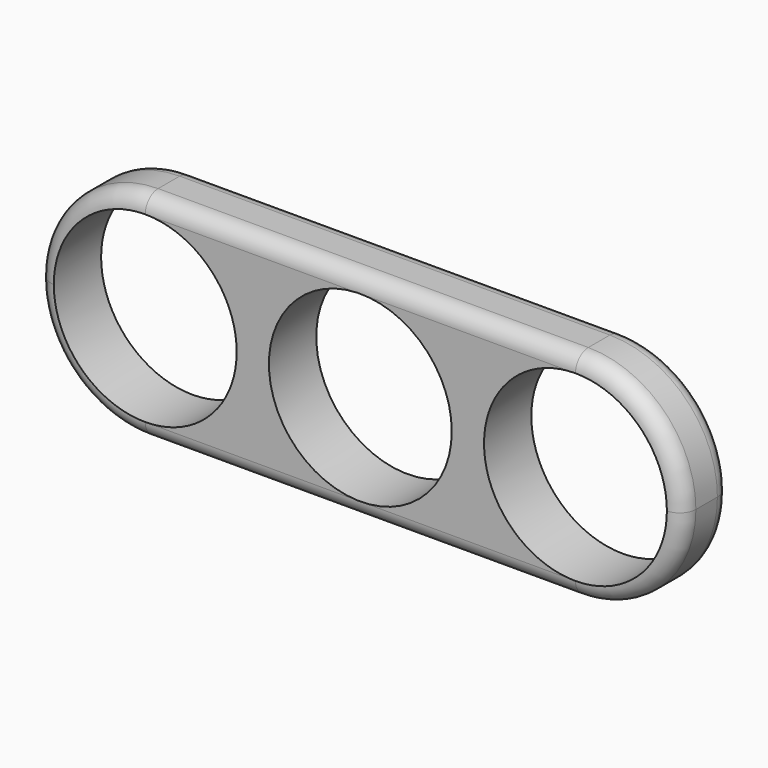
from build123d import *

# Parameters (mm, degrees)
F0_W     = 76.2
F0_H     = 25.4
F1_DEPTH = 6.985
F2_R     = 12.69999
F3_R     = 10.795
F4_DEPTH = 6.986
F5_R     = 1.90499


# Not quite as in the source:
# - a fillet or chamfer is up to 0.001 mm smaller than in the source, because OpenCascade refuses the exact size


with BuildPart() as f1:
    # F0 (on Front) → F1 (new body)
    with BuildSketch(Plane.XZ):
        with Locations((38.1, 12.7)):
            Rectangle(F0_W, F0_H)
    extrude(amount=F1_DEPTH)

    # F2 (radius 12.7 in the source; OpenCascade refuses exactly that, so slightly less here)
    f2_edges = [f1.edges().sort_by_distance(p)[0] for p in [
        (76.2, -3.4925, 25.4),
        (0, -3.4925, 25.4),
        (76.2, -3.4925, 0),
        (0, -3.4925, 0),
    ]]
    fillet(f2_edges, radius=F2_R)

    # F3 (on face) → F4 (cut, through all)
    with BuildSketch(Plane.XZ.offset(6.985)):
        with Locations((12.7, 12.7)):
            Circle(F3_R)
        with Locations((38.1, 12.7)):
            Circle(F3_R)
        with Locations((63.5, 12.7)):
            Circle(F3_R)
    extrude(amount=-F4_DEPTH, mode=Mode.SUBTRACT)

    # F5 (radius 1.905 in the source; OpenCascade refuses exactly that, so slightly less here)
    f5_edges = [f1.edges().sort_by_distance(p)[0] for p in [
        (38.1, -6.985, 25.4),
        (38.1, 0, 0),
    ]]
    fillet(f5_edges, radius=F5_R)


solid = f1.part
